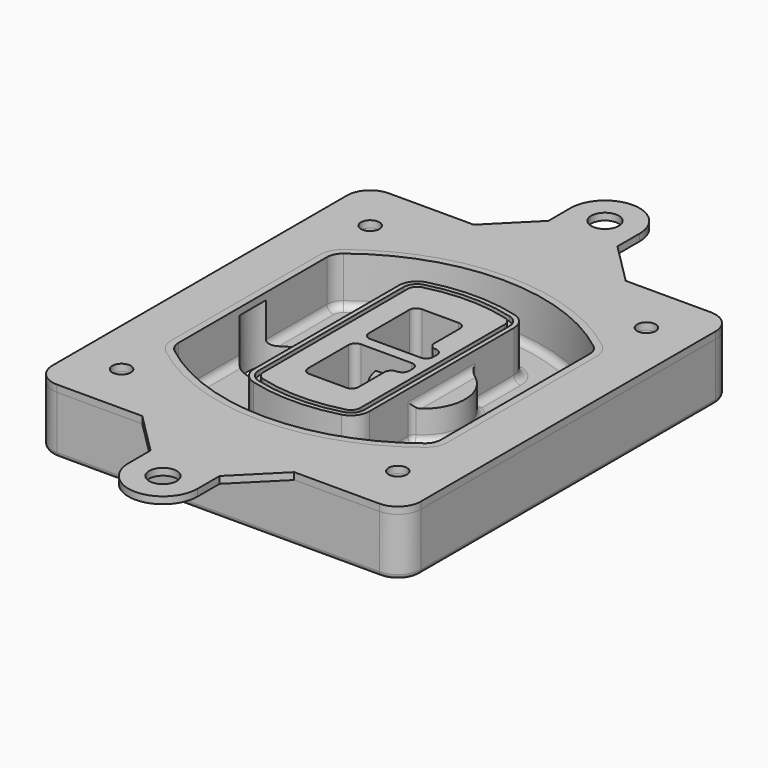
from build123d import *

# Parameters (mm, degrees)
F0_R      = 4
F1_DEPTH  = 25
F2_DEPTH  = 3
F3_DEPTH  = 18
F5_DEPTH  = 21
F6_DEPTH  = 2
F8_DEPTH  = 20
F9_DEPTH  = 16
F10_DEPTH = 25
F7_R      = 6
F7_R_2    = 4
F11_DEPTH = 6
F13_DEPTH = 9
F14_R     = 3
F15_R     = 2
F16_R     = 4
F16_R_2   = 6
F17_DEPTH = 3


# Not quite as in the source:
# - a feature names something its author has since deleted; it is built from what else it names


with BuildPart() as f1:
    # F0 (on Top) → F1 (new body)
    with BuildSketch(Plane.XY):
        with BuildLine():
            ThreePointArc((-80, -80), (-77.0710678119, -87.0710678119), (-70, -90))
            Line((-70, -90), (70, -90))
            ThreePointArc((70, -90), (77.0710678119, -87.0710678119), (80, -80))
            Line((80, -80), (80, 80))
            ThreePointArc((80, 80), (77.0710678119, 87.0710678119), (70, 90))
            Line((70, 90), (-70, 90))
            ThreePointArc((-70, 90), (-77.0710678119, 87.0710678119), (-80, 80))
            Line((-80, 80), (-80, -80))
        make_face()
        with Locations((-60, -67.5)):
            Circle(F0_R, mode=Mode.SUBTRACT)
        with Locations((60, -67.5)):
            Circle(F0_R, mode=Mode.SUBTRACT)
        with Locations((-60, 67.5)):
            Circle(F0_R, mode=Mode.SUBTRACT)
        with BuildLine():
            ThreePointArc((-64, 40.2934422872), (-62.5820384798, 46.4328484224), (-58.6153846154, 51.3286200352))
            ThreePointArc((-58.6153846154, 51.3286200352), (0, 71.5), (58.6153846154, 51.3286200352))
            ThreePointArc((58.6153846154, 51.3286200352), (62.5820384798, 46.4328484224), (64, 40.2934422872))
            Line((64, 40.2934422872), (64, -40.2934422872))
            ThreePointArc((64, -40.2934422872), (62.5820384798, -46.4328484224), (58.6153846154, -51.3286200352))
            ThreePointArc((58.6153846154, -51.3286200352), (0, -71.5), (-58.6153846154, -51.3286200352))
            ThreePointArc((-58.6153846154, -51.3286200352), (-62.5820384798, -46.4328484224), (-64, -40.2934422872))
            Line((-64, -40.2934422872), (-64, 40.2934422872))
        make_face(mode=Mode.SUBTRACT)
        with Locations((60, 67.5)):
            Circle(F0_R, mode=Mode.SUBTRACT)
        with BuildLine():
            ThreePointArc((58.6153846154, 51.3286200352), (0, 71.5), (-58.6153846154, 51.3286200352))
            ThreePointArc((-58.6153846154, 51.3286200352), (-62.5820384798, 46.4328484224), (-64, 40.2934422872))
            Line((-64, 40.2934422872), (-64, -40.2934422872))
            ThreePointArc((-64, -40.2934422872), (-62.5820384798, -46.4328484224), (-58.6153846154, -51.3286200352))
            ThreePointArc((-58.6153846154, -51.3286200352), (0, -71.5), (58.6153846154, -51.3286200352))
            ThreePointArc((58.6153846154, -51.3286200352), (62.5820384798, -46.4328484224), (64, -40.2934422872))
            Line((64, -40.2934422872), (64, 40.2934422872))
            ThreePointArc((64, 40.2934422872), (62.5820384798, 46.4328484224), (58.6153846154, 51.3286200352))
        make_face()
        with BuildLine():
            Line((-60, -40.2934422872), (-60, 40.2934422872))
            ThreePointArc((-60, 40.2934422872), (-58.9871703427, 44.6787323838), (-56.1538461538, 48.1757121072))
            ThreePointArc((-56.1538461538, 48.1757121072), (0, 67.5), (56.1538461538, 48.1757121072))
            ThreePointArc((56.1538461538, 48.1757121072), (58.9871703427, 44.6787323838), (60, 40.2934422872))
            Line((60, 40.2934422872), (60, -40.2934422872))
            ThreePointArc((60, -40.2934422872), (58.9871703427, -44.6787323838), (56.1538461538, -48.1757121072))
            ThreePointArc((56.1538461538, -48.1757121072), (0, -67.5), (-56.1538461538, -48.1757121072))
            ThreePointArc((-56.1538461538, -48.1757121072), (-58.9871703427, -44.6787323838), (-60, -40.2934422872))
        make_face(mode=Mode.SUBTRACT)
        with BuildLine():
            ThreePointArc((-56.1538461538, 48.1757121072), (-58.9871703427, 44.6787323838), (-60, 40.2934422872))
            Line((-60, 40.2934422872), (-60, -40.2934422872))
            ThreePointArc((-60, -40.2934422872), (-58.9871703427, -44.6787323838), (-56.1538461538, -48.1757121072))
            ThreePointArc((-56.1538461538, -48.1757121072), (0, -67.5), (56.1538461538, -48.1757121072))
            ThreePointArc((56.1538461538, -48.1757121072), (58.9871703427, -44.6787323838), (60, -40.2934422872))
            Line((60, -40.2934422872), (60, 40.2934422872))
            ThreePointArc((60, 40.2934422872), (58.9871703427, 44.6787323838), (56.1538461538, 48.1757121072))
            ThreePointArc((56.1538461538, 48.1757121072), (0, 67.5), (-56.1538461538, 48.1757121072))
        make_face()
        with BuildLine():
            ThreePointArc((54.3076923077, 45.8110311612), (56.2910192399, 43.3631453548), (57, 40.2934422872))
            Line((57, 40.2934422872), (57, -40.2934422872))
            ThreePointArc((57, -40.2934422872), (56.2910192399, -43.3631453548), (54.3076923077, -45.8110311612))
            ThreePointArc((54.3076923077, -45.8110311612), (0, -64.5), (-54.3076923077, -45.8110311612))
            ThreePointArc((-54.3076923077, -45.8110311612), (-56.2910192399, -43.3631453548), (-57, -40.2934422872))
            Line((-57, -40.2934422872), (-57, 40.2934422872))
            ThreePointArc((-57, 40.2934422872), (-56.2910192399, 43.3631453548), (-54.3076923077, 45.8110311612))
            ThreePointArc((-54.3076923077, 45.8110311612), (0, 64.5), (54.3076923077, 45.8110311612))
        make_face(mode=Mode.SUBTRACT)
        with BuildLine():
            Line((57, -40.2934422872), (57, 40.2934422872))
            ThreePointArc((57, 40.2934422872), (56.2910192399, 43.3631453548), (54.3076923077, 45.8110311612))
            ThreePointArc((54.3076923077, 45.8110311612), (0, 64.5), (-54.3076923077, 45.8110311612))
            ThreePointArc((-54.3076923077, 45.8110311612), (-56.2910192399, 43.3631453548), (-57, 40.2934422872))
            Line((-57, 40.2934422872), (-57, -40.2934422872))
            ThreePointArc((-57, -40.2934422872), (-56.2910192399, -43.3631453548), (-54.3076923077, -45.8110311612))
            ThreePointArc((-54.3076923077, -45.8110311612), (0, -64.5), (54.3076923077, -45.8110311612))
            ThreePointArc((54.3076923077, -45.8110311612), (56.2910192399, -43.3631453548), (57, -40.2934422872))
        make_face()
    extrude(amount=-F1_DEPTH)

    # F0 (on Top) → F2 (join)
    with BuildSketch(Plane.XY):
        with BuildLine():
            ThreePointArc((-56.1538461538, 48.1757121072), (-58.9871703427, 44.6787323838), (-60, 40.2934422872))
            Line((-60, 40.2934422872), (-60, -40.2934422872))
            ThreePointArc((-60, -40.2934422872), (-58.9871703427, -44.6787323838), (-56.1538461538, -48.1757121072))
            ThreePointArc((-56.1538461538, -48.1757121072), (0, -67.5), (56.1538461538, -48.1757121072))
            ThreePointArc((56.1538461538, -48.1757121072), (58.9871703427, -44.6787323838), (60, -40.2934422872))
            Line((60, -40.2934422872), (60, 40.2934422872))
            ThreePointArc((60, 40.2934422872), (58.9871703427, 44.6787323838), (56.1538461538, 48.1757121072))
            ThreePointArc((56.1538461538, 48.1757121072), (0, 67.5), (-56.1538461538, 48.1757121072))
        make_face()
        with BuildLine():
            ThreePointArc((54.3076923077, 45.8110311612), (56.2910192399, 43.3631453548), (57, 40.2934422872))
            Line((57, 40.2934422872), (57, -40.2934422872))
            ThreePointArc((57, -40.2934422872), (56.2910192399, -43.3631453548), (54.3076923077, -45.8110311612))
            ThreePointArc((54.3076923077, -45.8110311612), (0, -64.5), (-54.3076923077, -45.8110311612))
            ThreePointArc((-54.3076923077, -45.8110311612), (-56.2910192399, -43.3631453548), (-57, -40.2934422872))
            Line((-57, -40.2934422872), (-57, 40.2934422872))
            ThreePointArc((-57, 40.2934422872), (-56.2910192399, 43.3631453548), (-54.3076923077, 45.8110311612))
            ThreePointArc((-54.3076923077, 45.8110311612), (0, 64.5), (54.3076923077, 45.8110311612))
        make_face(mode=Mode.SUBTRACT)
    extrude(amount=F2_DEPTH)

    # F0 (on Top) → F3 (cut)
    with BuildSketch(Plane.XY):
        with BuildLine():
            Line((57, -40.2934422872), (57, 40.2934422872))
            ThreePointArc((57, 40.2934422872), (56.2910192399, 43.3631453548), (54.3076923077, 45.8110311612))
            ThreePointArc((54.3076923077, 45.8110311612), (0, 64.5), (-54.3076923077, 45.8110311612))
            ThreePointArc((-54.3076923077, 45.8110311612), (-56.2910192399, 43.3631453548), (-57, 40.2934422872))
            Line((-57, 40.2934422872), (-57, -40.2934422872))
            ThreePointArc((-57, -40.2934422872), (-56.2910192399, -43.3631453548), (-54.3076923077, -45.8110311612))
            ThreePointArc((-54.3076923077, -45.8110311612), (0, -64.5), (54.3076923077, -45.8110311612))
            ThreePointArc((54.3076923077, -45.8110311612), (56.2910192399, -43.3631453548), (57, -40.2934422872))
        make_face()
    extrude(amount=-F3_DEPTH, mode=Mode.SUBTRACT)

    # F4 (on face) → F5 (join, through all)
    with BuildSketch(Plane.XY.offset(3)):
        with BuildLine():
            ThreePointArc((-25, -39.2465276821), (-23.3511545998, -44.1109737193), (-19.0842911877, -46.9702398883))
            ThreePointArc((-19.0842911877, -46.9702398883), (0, -49.5), (19.0842911877, -46.9702398883))
            ThreePointArc((19.0842911877, -46.9702398883), (23.3511545998, -44.1109737193), (25, -39.2465276821))
            Line((25, -39.2465276821), (25, 39.2465276821))
            ThreePointArc((25, 39.2465276821), (23.3511545998, 44.1109737193), (19.0842911877, 46.9702398883))
            ThreePointArc((19.0842911877, 46.9702398883), (0, 49.5), (-19.0842911877, 46.9702398883))
            ThreePointArc((-19.0842911877, 46.9702398883), (-23.3511545998, 44.1109737193), (-25, 39.2465276821))
            Line((-25, 39.2465276821), (-25, -39.2465276821))
        make_face()
        with BuildLine():
            ThreePointArc((18.5632183908, 45.0393118368), (21.7633659499, 42.89486221), (23, 39.2465276821))
            Line((23, 39.2465276821), (23, -39.2465276821))
            ThreePointArc((23, -39.2465276821), (21.7633659499, -42.89486221), (18.5632183908, -45.0393118368))
            ThreePointArc((18.5632183908, -45.0393118368), (0, -47.5), (-18.5632183908, -45.0393118368))
            ThreePointArc((-18.5632183908, -45.0393118368), (-21.7633659499, -42.89486221), (-23, -39.2465276821))
            Line((-23, -39.2465276821), (-23, 39.2465276821))
            ThreePointArc((-23, 39.2465276821), (-21.7633659499, 42.89486221), (-18.5632183908, 45.0393118368))
            ThreePointArc((-18.5632183908, 45.0393118368), (0, 47.5), (18.5632183908, 45.0393118368))
        make_face(mode=Mode.SUBTRACT)
        with BuildLine():
            Line((23, -39.2465276821), (23, 39.2465276821))
            ThreePointArc((23, 39.2465276821), (21.7633659499, 42.89486221), (18.5632183908, 45.0393118368))
            ThreePointArc((18.5632183908, 45.0393118368), (0, 47.5), (-18.5632183908, 45.0393118368))
            ThreePointArc((-18.5632183908, 45.0393118368), (-21.7633659499, 42.89486221), (-23, 39.2465276821))
            Line((-23, 39.2465276821), (-23, -39.2465276821))
            ThreePointArc((-23, -39.2465276821), (-21.7633659499, -42.89486221), (-18.5632183908, -45.0393118368))
            ThreePointArc((-18.5632183908, -45.0393118368), (0, -47.5), (18.5632183908, -45.0393118368))
            ThreePointArc((18.5632183908, -45.0393118368), (21.7633659499, -42.89486221), (23, -39.2465276821))
        make_face()
        with BuildLine():
            ThreePointArc((18.0421455939, 43.1083837852), (20.1755772999, 41.6787507007), (21, 39.2465276821))
            Line((21, 39.2465276821), (21, -39.2465276821))
            ThreePointArc((21, -39.2465276821), (20.1755772999, -41.6787507007), (18.0421455939, -43.1083837852))
            ThreePointArc((18.0421455939, -43.1083837852), (0, -45.5), (-18.0421455939, -43.1083837852))
            ThreePointArc((-18.0421455939, -43.1083837852), (-20.1755772999, -41.6787507007), (-21, -39.2465276821))
            Line((-21, -39.2465276821), (-21, 39.2465276821))
            ThreePointArc((-21, 39.2465276821), (-20.1755772999, 41.6787507007), (-18.0421455939, 43.1083837852))
            ThreePointArc((-18.0421455939, 43.1083837852), (0, 45.5), (18.0421455939, 43.1083837852))
        make_face(mode=Mode.SUBTRACT)
        with BuildLine():
            Line((21, -39.2465276821), (21, 39.2465276821))
            ThreePointArc((21, 39.2465276821), (20.1755772999, 41.6787507007), (18.0421455939, 43.1083837852))
            ThreePointArc((18.0421455939, 43.1083837852), (0, 45.5), (-18.0421455939, 43.1083837852))
            ThreePointArc((-18.0421455939, 43.1083837852), (-20.1755772999, 41.6787507007), (-21, 39.2465276821))
            Line((-21, 39.2465276821), (-21, -39.2465276821))
            ThreePointArc((-21, -39.2465276821), (-20.1755772999, -41.6787507007), (-18.0421455939, -43.1083837852))
            ThreePointArc((-18.0421455939, -43.1083837852), (0, -45.5), (18.0421455939, -43.1083837852))
            ThreePointArc((18.0421455939, -43.1083837852), (20.1755772999, -41.6787507007), (21, -39.2465276821))
        make_face()
        with BuildLine():
            Line((-8, -2.5), (14, -2.5))
            ThreePointArc((14, -2.5), (16.1213203436, -3.3786796564), (17, -5.5))
            Line((17, -5.5), (17, -7.5))
            ThreePointArc((17, -7.5), (16.1213203436, -9.6213203436), (14, -10.5))
            ThreePointArc((14, -10.5), (11.8786796564, -11.3786796564), (11, -13.5))
            Line((11, -13.5), (11, -27.5))
            ThreePointArc((11, -27.5), (10.1213203436, -29.6213203436), (8, -30.5))
            Line((8, -30.5), (-8, -30.5))
            ThreePointArc((-8, -30.5), (-10.1213203436, -29.6213203436), (-11, -27.5))
            Line((-11, -27.5), (-11, -5.5))
            ThreePointArc((-11, -5.5), (-10.1213203436, -3.3786796564), (-8, -2.5))
        make_face(mode=Mode.SUBTRACT)
        with BuildLine():
            ThreePointArc((-8, 2.5), (-10.1213203436, 3.3786796564), (-11, 5.5))
            Line((-11, 5.5), (-11, 27.5))
            ThreePointArc((-11, 27.5), (-10.1213203436, 29.6213203436), (-8, 30.5))
            Line((-8, 30.5), (8, 30.5))
            ThreePointArc((8, 30.5), (10.1213203436, 29.6213203436), (11, 27.5))
            Line((11, 27.5), (11, 13.5))
            ThreePointArc((11, 13.5), (11.8786796564, 11.3786796564), (14, 10.5))
            ThreePointArc((14, 10.5), (16.1213203436, 9.6213203436), (17, 7.5))
            Line((17, 7.5), (17, 5.5))
            ThreePointArc((17, 5.5), (16.1213203436, 3.3786796564), (14, 2.5))
            Line((14, 2.5), (-8, 2.5))
        make_face(mode=Mode.SUBTRACT)
    extrude(amount=-F5_DEPTH)

    # F4 (on face) → F6 (cut)
    with BuildSketch(Plane.XY.offset(3)):
        with BuildLine():
            Line((23, -39.2465276821), (23, 39.2465276821))
            ThreePointArc((23, 39.2465276821), (21.7633659499, 42.89486221), (18.5632183908, 45.0393118368))
            ThreePointArc((18.5632183908, 45.0393118368), (0, 47.5), (-18.5632183908, 45.0393118368))
            ThreePointArc((-18.5632183908, 45.0393118368), (-21.7633659499, 42.89486221), (-23, 39.2465276821))
            Line((-23, 39.2465276821), (-23, -39.2465276821))
            ThreePointArc((-23, -39.2465276821), (-21.7633659499, -42.89486221), (-18.5632183908, -45.0393118368))
            ThreePointArc((-18.5632183908, -45.0393118368), (0, -47.5), (18.5632183908, -45.0393118368))
            ThreePointArc((18.5632183908, -45.0393118368), (21.7633659499, -42.89486221), (23, -39.2465276821))
        make_face()
        with BuildLine():
            ThreePointArc((18.0421455939, 43.1083837852), (20.1755772999, 41.6787507007), (21, 39.2465276821))
            Line((21, 39.2465276821), (21, -39.2465276821))
            ThreePointArc((21, -39.2465276821), (20.1755772999, -41.6787507007), (18.0421455939, -43.1083837852))
            ThreePointArc((18.0421455939, -43.1083837852), (0, -45.5), (-18.0421455939, -43.1083837852))
            ThreePointArc((-18.0421455939, -43.1083837852), (-20.1755772999, -41.6787507007), (-21, -39.2465276821))
            Line((-21, -39.2465276821), (-21, 39.2465276821))
            ThreePointArc((-21, 39.2465276821), (-20.1755772999, 41.6787507007), (-18.0421455939, 43.1083837852))
            ThreePointArc((-18.0421455939, 43.1083837852), (0, 45.5), (18.0421455939, 43.1083837852))
        make_face(mode=Mode.SUBTRACT)
    extrude(amount=-F6_DEPTH, mode=Mode.SUBTRACT)

    # F7 (on face) → F8 (join)
    with BuildSketch(Plane(origin=(0, 0, -25), x_dir=(1, 0, 0), z_dir=(0, 0, -1))):
        with BuildLine():
            ThreePointArc((3.28842436, 0), (16.7567035675, 13.4682792075), (30.224982775, 0))
            Line((30.224982775, 0), (35.224982775, 0))
            ThreePointArc((35.224982775, 0), (16.7567035675, 18.4682792075), (-1.71157564, 0))
            Line((-1.71157564, 0), (3.28842436, 0))
        make_face()
        with BuildLine():
            Line((3.28842436, 0), (30.224982775, 0))
            ThreePointArc((30.224982775, 0), (16.7567035675, 13.4682792075), (3.28842436, 0))
        make_face()
        with BuildLine():
            ThreePointArc((3.28842436, 0), (16.7567035675, -13.4682792075), (30.224982775, 0))
            Line((30.224982775, 0), (3.28842436, 0))
        make_face()
        with BuildLine():
            Line((35.224982775, 0), (30.224982775, 0))
            ThreePointArc((30.224982775, 0), (16.7567035675, -13.4682792075), (3.28842436, 0))
            Line((3.28842436, 0), (-1.71157564, 0))
            ThreePointArc((-1.71157564, 0), (16.7567035675, -18.4682792075), (35.224982775, 0))
        make_face()
    extrude(amount=-F8_DEPTH)

    # F7 (on face) → F9 (cut)
    with BuildSketch(Plane(origin=(0, 0, -25), x_dir=(1, 0, 0), z_dir=(0, 0, -1))):
        with BuildLine():
            Line((3.28842436, 0), (30.224982775, 0))
            ThreePointArc((30.224982775, 0), (16.7567035675, 13.4682792075), (3.28842436, 0))
        make_face()
        with BuildLine():
            ThreePointArc((3.28842436, 0), (16.7567035675, -13.4682792075), (30.224982775, 0))
            Line((30.224982775, 0), (3.28842436, 0))
        make_face()
    extrude(amount=-F9_DEPTH, mode=Mode.SUBTRACT)

    # F7 (on face) → F10 (cut)
    with BuildSketch(Plane(origin=(0, 0, -25), x_dir=(1, 0, 0), z_dir=(0, 0, -1))):
        with BuildLine():
            Line((-59.0318229325, 0), (-32.0952645175, 0))
            ThreePointArc((-32.0952645175, 0), (-45.563543725, 13.4682792075), (-59.0318229325, 0))
        make_face()
        with BuildLine():
            ThreePointArc((-59.0318229325, 0), (-45.563543725, -13.4682792075), (-32.0952645175, 0))
            Line((-32.0952645175, 0), (-59.0318229325, 0))
        make_face()
    extrude(amount=-F10_DEPTH, mode=Mode.SUBTRACT)

    # F7 (on face) → F11 (cut)
    with BuildSketch(Plane(origin=(0, 0, -25), x_dir=(1, 0, 0), z_dir=(0, 0, -1))):
        with Locations((60, -67.5)):
            Circle(F7_R)
        with Locations((60, -67.5)):
            Circle(F7_R_2, mode=Mode.SUBTRACT)
        with Locations((-60, -67.5)):
            Circle(F7_R)
        with Locations((-60, -67.5)):
            Circle(F7_R_2, mode=Mode.SUBTRACT)
        with Locations((-60, 67.5)):
            Circle(F7_R)
        with Locations((-60, 67.5)):
            Circle(F7_R_2, mode=Mode.SUBTRACT)
        with Locations((60, 67.5)):
            Circle(F7_R)
        with Locations((60, 67.5)):
            Circle(F7_R_2, mode=Mode.SUBTRACT)
    extrude(amount=-F11_DEPTH, mode=Mode.SUBTRACT)

    # F12 (on face) → F13 (cut, through all)
    with BuildSketch(Plane(origin=(0, 0, -9), x_dir=(1, 0, 0), z_dir=(0, 0, -1))):
        with BuildLine():
            Line((11, 13.5), (11, 17.5481537753))
            ThreePointArc((11, 17.5481537753), (2.5696536419, 11.8239143813), (-1.5415842455, 2.5))
            Line((-1.5415842455, 2.5), (3.5224848595, 2.5))
            ThreePointArc((3.5224848595, 2.5), (6.1857188154, 8.3455872281), (11.2536447004, 12.2927168648))
            ThreePointArc((11.2536447004, 12.2927168648), (11.0640958889, 12.8831798879), (11, 13.5))
        make_face()
        with BuildLine():
            ThreePointArc((11.2536447004, -12.2927168648), (6.1857188154, -8.3455872281), (3.5224848595, -2.5))
            Line((3.5224848595, -2.5), (-1.5415842455, -2.5))
            ThreePointArc((-1.5415842455, -2.5), (2.5696536419, -11.8239143813), (11, -17.5481537753))
            Line((11, -17.5481537753), (11, -13.5))
            ThreePointArc((11, -13.5), (11.0640958889, -12.8831798879), (11.2536447004, -12.2927168648))
        make_face()
        with BuildLine():
            ThreePointArc((11.2536447004, 12.2927168648), (6.1857188154, 8.3455872281), (3.5224848595, 2.5))
            Line((3.5224848595, 2.5), (14, 2.5))
            ThreePointArc((14, 2.5), (16.1213203436, 3.3786796564), (17, 5.5))
            Line((17, 5.5), (17, 7.5))
            ThreePointArc((17, 7.5), (16.1213203436, 9.6213203436), (14, 10.5))
            ThreePointArc((14, 10.5), (12.3601599782, 10.9878446101), (11.2536447004, 12.2927168648))
        make_face()
        with BuildLine():
            Line((14, -2.5), (3.5224848595, -2.5))
            ThreePointArc((3.5224848595, -2.5), (6.1857188154, -8.3455872281), (11.2536447004, -12.2927168648))
            ThreePointArc((11.2536447004, -12.2927168648), (12.3601599782, -10.9878446101), (14, -10.5))
            ThreePointArc((14, -10.5), (16.1213203436, -9.6213203436), (17, -7.5))
            Line((17, -7.5), (17, -5.5))
            ThreePointArc((17, -5.5), (16.1213203436, -3.3786796564), (14, -2.5))
        make_face()
    extrude(amount=F13_DEPTH, mode=Mode.SUBTRACT)

    # F14
    f14_edges = [f1.edges().sort_by_distance(p)[0] for p in [
        (-57, -23.703476, -18),
        (-57, 23.703476, -18),
        (25, 0, -5),
        (25, 16.526506, -11.5),
        (25, -16.526506, -11.5),
        (25, -27.886517, -18),
        (35.224983, 0, -18),
    ]]
    fillet(f14_edges, radius=F14_R)

    # F15
    f15_edges = [f1.edges().sort_by_distance(p)[0] for p in [
        (0, -90, -25),
    ]]
    fillet(f15_edges, radius=F15_R)


with BuildPart() as f17:
    # F16 (on face) → F17 (new body, through all)
    with BuildSketch(Plane.XY):
        with BuildLine():
            Line((-33, 90), (-70, 90))
            ThreePointArc((-70, 90), (-77.0710678119, 87.0710678119), (-80, 80))
            Line((-80, 80), (-80, -80))
            ThreePointArc((-80, -80), (-77.0710678119, -87.0710678119), (-70, -90))
            Line((-70, -90), (-33, -90))
            Line((-33, -90), (33, -90))
            Line((33, -90), (70, -90))
            ThreePointArc((70, -90), (77.0710678119, -87.0710678119), (80, -80))
            Line((80, -80), (80, 80))
            ThreePointArc((80, 80), (77.0710678119, 87.0710678119), (70, 90))
            Line((70, 90), (33, 90))
            Line((33, 90), (-33, 90))
        make_face()
        with Locations((-60, -67.5)):
            Circle(F16_R, mode=Mode.SUBTRACT)
        with Locations((60, -67.5)):
            Circle(F16_R, mode=Mode.SUBTRACT)
        with Locations((-60, 67.5)):
            Circle(F16_R, mode=Mode.SUBTRACT)
        with BuildLine():
            ThreePointArc((56.1538461538, -48.1757121072), (0, -67.5), (-56.1538461538, -48.1757121072))
            ThreePointArc((-56.1538461538, -48.1757121072), (-58.9871703427, -44.6787323838), (-60, -40.2934422872))
            Line((-60, -40.2934422872), (-60, 40.2934422872))
            ThreePointArc((-60, 40.2934422872), (-58.9871703427, 44.6787323838), (-56.1538461538, 48.1757121072))
            ThreePointArc((-56.1538461538, 48.1757121072), (0, 67.5), (56.1538461538, 48.1757121072))
            ThreePointArc((56.1538461538, 48.1757121072), (58.9871703427, 44.6787323838), (60, 40.2934422872))
            Line((60, 40.2934422872), (60, -40.2934422872))
            ThreePointArc((60, -40.2934422872), (58.9871703427, -44.6787323838), (56.1538461538, -48.1757121072))
        make_face(mode=Mode.SUBTRACT)
        with Locations((60, 67.5)):
            Circle(F16_R, mode=Mode.SUBTRACT)
        with BuildLine():
            Line((33, -90), (-33, -90))
            Line((-33, -90), (-15, -108))
            Line((-15, -108), (-15, -120))
            ThreePointArc((-15, -120), (0, -135), (15, -120))
            Line((15, -120), (15, -108))
            Line((15, -108), (33, -90))
        make_face()
        with Locations((0, -120)):
            Circle(F16_R_2, mode=Mode.SUBTRACT)
        with BuildLine():
            Line((-15, 108), (-33, 90))
            Line((-33, 90), (33, 90))
            Line((33, 90), (15, 108))
            Line((15, 108), (15, 120))
            ThreePointArc((15, 120), (0, 135), (-15, 120))
            Line((-15, 120), (-15, 108))
        make_face()
        with Locations((0, 120)):
            Circle(F16_R_2, mode=Mode.SUBTRACT)
    extrude(amount=F17_DEPTH)


solid = Compound([f1.part, f17.part])
